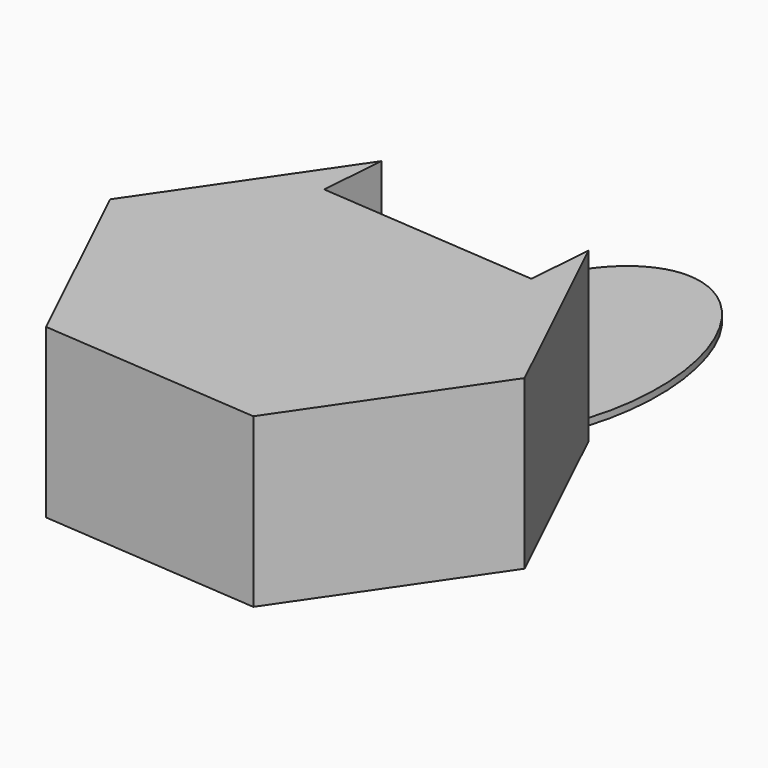
from build123d import *

# Parameters (mm, degrees)
F2_DEPTH = 25.4
F4_DEPTH = 9.906
F6_DEPTH = 1.016


# Not quite as in the source:
# - the program builds the solid bodies; features that only make, move or delete a surface that nothing else refers to are left out


with BuildPart() as f2:
    # F0 (on Top) → F2 (new body)
    with BuildSketch(Plane.XY):
        Polygon((-98.1804851865, 42.2748850128), (-83.6932088757, 12.0514331916), (-50.2752936531, 9.4860565979), (-31.3446547413, 37.1441318253), (-45.8319310522, 67.3675836465), (-79.2498462748, 69.9329602402), align=None)
    extrude(amount=F2_DEPTH)

    # F4 (cut): a face of the model
    f4_faces = [f2.faces().sort_by_distance(p)[0] for p in [
        (-62.5408886635, 68.6502719433, 12.7),
    ]]
    extrude(f4_faces, amount=-F4_DEPTH, mode=Mode.SUBTRACT)

    # F5 (on Top) → F6 (join)
    with BuildSketch(Plane.XY):
        with BuildLine():
            add(Edge.make_bspline(
                [(-63.3374005556, 107.8479960561), (-90.0996928702, 107.8479960561), (-76.7185467129, 70.8282925189), (-63.3374005556, 33.8085889816), (-49.9562543983, 70.8282925189), (-36.575108241, 107.8479960561), (-63.3374005556, 107.8479960561)],
                knots=[0, 0, 0, 2.0943951024, 2.0943951024, 4.1887902048, 4.1887902048, 6.2831853072, 6.2831853072, 6.2831853072], degree=2, weights=[1, 0.5, 1, 0.5, 1, 0.5, 1]))
        make_face()
    extrude(amount=-F6_DEPTH)


solid = f2.part
